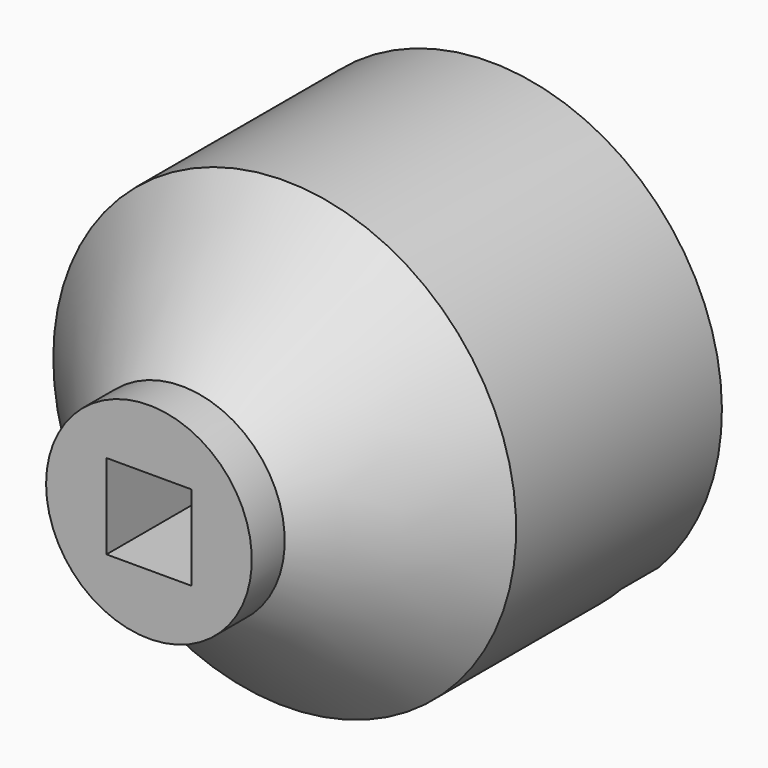
from build123d import *

# Parameters (mm, degrees)
F0_W     = 10
F0_H     = 4
F0_W_2   = 22.5
F0_H_2   = 25
F2_W     = 8.25
F2_H     = 8.25
F3_DEPTH = 41.501
F2_W_2   = 13.25
F2_H_2   = 25
F4_DEPTH = 6
F2_W_3   = 6.375
F5_DEPTH = 4.5
F6_R     = 2
F8_W     = 6.5
F8_H     = 6.5
F9_DEPTH = 25


with BuildPart() as f1:
    # F0 (on Top) → F1 (revolve)
    with BuildSketch(Plane.XY):
        with Locations((-5, -27)):
            Rectangle(F0_W, F0_H)
        Polygon((0, -25), (0, -12.5), (-22.5, -12.5), (-10, -25), align=None)
        with Locations((-11.25, 0)):
            Rectangle(F0_W_2, F0_H_2)
    revolve(axis=Axis((0, -8.25, 0), (0, -1, 0)))

    # F2 (on face) → F3 (cut, through all)
    with BuildSketch(Plane(origin=(0, 12.5, 0), x_dir=(-1, 0, 0), z_dir=(0, 1, 0))):
        Rectangle(F2_W, F2_H)
    extrude(amount=-F3_DEPTH, mode=Mode.SUBTRACT)

    # F2 (on face) → F4 (cut)
    with BuildSketch(Plane(origin=(0, 12.5, 0), x_dir=(-1, 0, 0), z_dir=(0, 1, 0))):
        Rectangle(F2_W_2, F2_H_2)
        Rectangle(F2_W, F2_H, mode=Mode.SUBTRACT)
    extrude(amount=-F4_DEPTH, mode=Mode.SUBTRACT)

    # F2 (on face) → F5 (cut)
    with BuildSketch(Plane(origin=(0, 12.5, 0), x_dir=(-1, 0, 0), z_dir=(0, 1, 0))):
        with BuildLine():
            Line((13, -18.3643676722), (13, -12.5))
            Line((13, -12.5), (6.625, -12.5))
            Line((6.625, -12.5), (-6.625, -12.5))
            Line((-6.625, -12.5), (-13, -12.5))
            Line((-13, -12.5), (-13, -18.3643676722))
            ThreePointArc((-13, -18.3643676722), (-6.8209870025, -21.4411785197), (0, -22.5))
            ThreePointArc((0, -22.5), (6.8209870025, -21.4411785197), (13, -18.3643676722))
        make_face()
        with Locations((9.8125, 0)):
            Rectangle(F2_W_3, F2_H_2)
        Rectangle(F2_W_2, F2_H_2)
        Rectangle(F2_W, F2_H, mode=Mode.SUBTRACT)
        with Locations((-9.8125, 0)):
            Rectangle(F2_W_3, F2_H_2)
    extrude(amount=-F5_DEPTH, mode=Mode.SUBTRACT)

    # F6
    f6_edges = [f1.edges().sort_by_distance(p)[0] for p in [
        (13, 10.25, -18.364368),
        (-13, 10.25, -18.364368),
    ]]
    fillet(f6_edges, radius=F6_R)

    # F8 (on offset) → F9 (cut)
    with BuildSketch(Plane.XY.offset(-25)):
        with Locations((0, -1.25)):
            Rectangle(F8_W, F8_H)
    extrude(amount=F9_DEPTH, mode=Mode.SUBTRACT)


solid = f1.part
